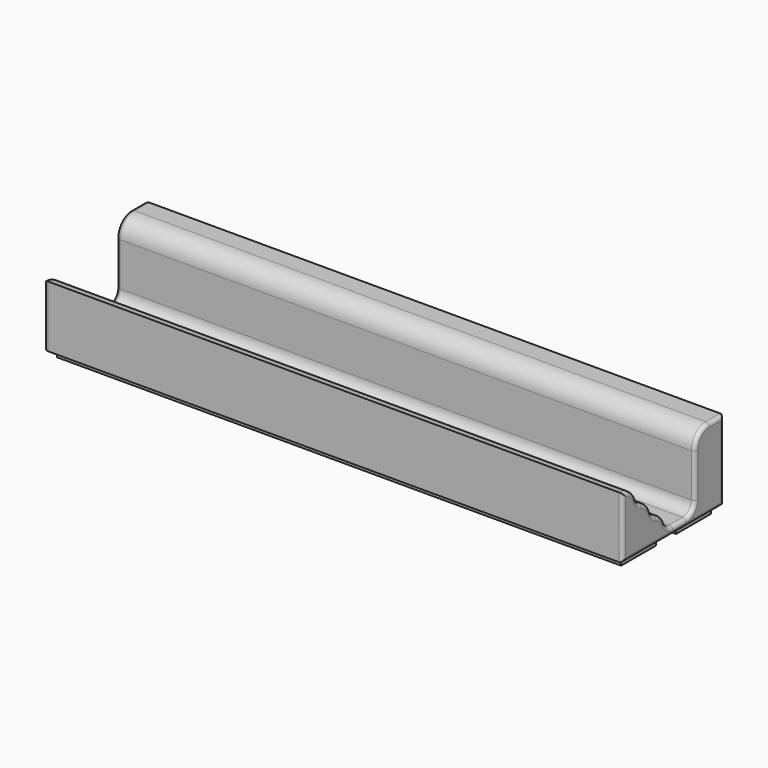
from build123d import *

# Parameters (mm, degrees)
F1_DEPTH  = 80
F2_W      = 156
F2_H      = 31
F3_DEPTH  = 2
F4_W      = 5
F4_H      = 5
F5_DEPTH  = 2.2
F6_W      = 5
F6_H      = 7
F7_DEPTH  = 2
F8_W      = 5
F8_H      = 3
F9_DEPTH  = 4.2
F10_R     = 1.99999
F11_W     = 20
F11_H     = 7
F12_DEPTH = 2
F13_R     = 3
F14_R     = 0.99999


# Not quite as in the source:
# - a fillet or chamfer is up to 0.001 mm smaller than in the source, because OpenCascade refuses the exact size


with BuildPart() as f1:
    # F0 (on Right) → F1 (new body, symmetric)
    with BuildSketch(Plane.YZ):
        with BuildLine():
            Line((7.5, 1), (17.5, 1))
            Line((17.5, 1), (17.5, 21))
            Line((17.5, 21), (12.5, 21))
            ThreePointArc((12.5, 21), (8.9644660941, 19.5355339059), (7.5, 16))
            Line((7.5, 16), (7.5, 1))
        make_face()
        Polygon((17.5, -1), (17.5, 1), (7.5, 1), (-2.5, 1), (-7.5, 1), (-12.5, 1), (-17.5, 1), (-17.5, -1), align=None)
        with BuildLine():
            Line((-17.5, 16), (-17.5, 1))
            Line((-17.5, 1), (-12.5, 1))
            Line((-12.5, 1), (-12.5, 11))
            ThreePointArc((-12.5, 11), (-13.9644660941, 14.5355339059), (-17.5, 16))
        make_face()
        with BuildLine():
            Line((-12.5, 1), (-7.5, 1))
            Line((-7.5, 1), (-7.5, 6))
            ThreePointArc((-7.5, 6), (-8.9644660941, 9.5355339059), (-12.5, 11))
            Line((-12.5, 11), (-12.5, 1))
        make_face()
        with BuildLine():
            Line((-7.5, 1), (-2.5, 1))
            ThreePointArc((-2.5, 1), (-3.9644660941, 4.5355339059), (-7.5, 6))
            Line((-7.5, 6), (-7.5, 1))
        make_face()
    extrude(amount=F1_DEPTH, both=True)

    # F2 (on face) → F3 (join)
    with BuildSketch(Plane(origin=(0, 0, -1), x_dir=(1, 0, 0), z_dir=(0, 0, -1))):
        Rectangle(F2_W, F2_H)
    extrude(amount=F3_DEPTH)

    # F4 (on face) → F5 (join)
    with BuildSketch(Plane(origin=(0, 0, -3), x_dir=(1, 0, 0), z_dir=(0, 0, -1))):
        with Locations((38, 0)):
            Rectangle(F4_W, F4_H)
    extrude(amount=F5_DEPTH)

    # F6 (on face) → F7 (join)
    with BuildSketch(Plane(origin=(0, 0, -5.2), x_dir=(1, 0, 0), z_dir=(0, 0, -1))):
        with Locations((38, 0)):
            Rectangle(F6_W, F6_H)
    extrude(amount=F7_DEPTH)

    # F8 (on face) → F9 (cut)
    with BuildSketch(Plane(origin=(0, 0, -7.2), x_dir=(1, 0, 0), z_dir=(0, 0, -1))):
        with Locations((38, 0)):
            Rectangle(F8_W, F8_H)
    extrude(amount=-F9_DEPTH, mode=Mode.SUBTRACT)

    # F10 (radius 2 in the source; OpenCascade refuses exactly that, so slightly less here)
    f10_edges = [f1.edges().sort_by_distance(p)[0] for p in [
        (40.5, 2.5, -7.2),
        (38, 3.5, -7.2),
        (40.5, -2.5, -7.2),
        (38, -3.5, -7.2),
        (35.5, -2.5, -7.2),
        (35.5, 2.5, -7.2),
    ]]
    fillet(f10_edges, radius=F10_R)

    # F11 (on face) → F12 (cut)
    with BuildSketch(Plane(origin=(0, 0, -3), x_dir=(1, 0, 0), z_dir=(0, 0, -1))):
        with Locations((68, 0)):
            Rectangle(F11_W, F11_H)
    extrude(amount=-F12_DEPTH, mode=Mode.SUBTRACT)

    # F13
    f13_edges = [f1.edges().sort_by_distance(p)[0] for p in [
        (0, -12.5, 11),
        (0, -7.5, 6),
        (0, -2.5, 1),
        (0, 7.5, 1),
    ]]
    fillet(f13_edges, radius=F13_R)

    # F14 (radius 1 in the source; OpenCascade refuses exactly that, so slightly less here)
    f14_edges = [f1.edges().sort_by_distance(p)[0] for p in [
        (80, 7.5, 10),
        (80, 6.62132, 1.87868),
        (80, 8.964466, 19.535534),
        (80, 2.208099, 1),
        (80, 15, 21),
        (80, -1.760852, 1.512531),
        (80, 17.5, 10),
        (80, -4.066216, 4.634436),
        (80, 0, -1),
        (80, -7.046875, 6.453125),
        (80, -17.5, 7.5),
        (80, -8.964466, 9.535534),
        (80, -14.588398, 15.064797),
        (80, -12.046875, 11.453125),
        (-80, 7.5, 10),
        (-80, 6.62132, 1.87868),
        (-80, 8.964466, 19.535534),
        (-80, 2.208099, 1),
        (-80, 15, 21),
        (-80, -1.760852, 1.512531),
        (-80, 17.5, 10),
        (-80, -4.066216, 4.634436),
        (-80, 0, -1),
        (-80, -7.046875, 6.453125),
        (-80, -17.5, 7.5),
        (-80, -8.964466, 9.535534),
        (-80, -14.588398, 15.064797),
        (-80, -12.046875, 11.453125),
    ]]
    fillet(f14_edges, radius=F14_R)


solid = f1.part
